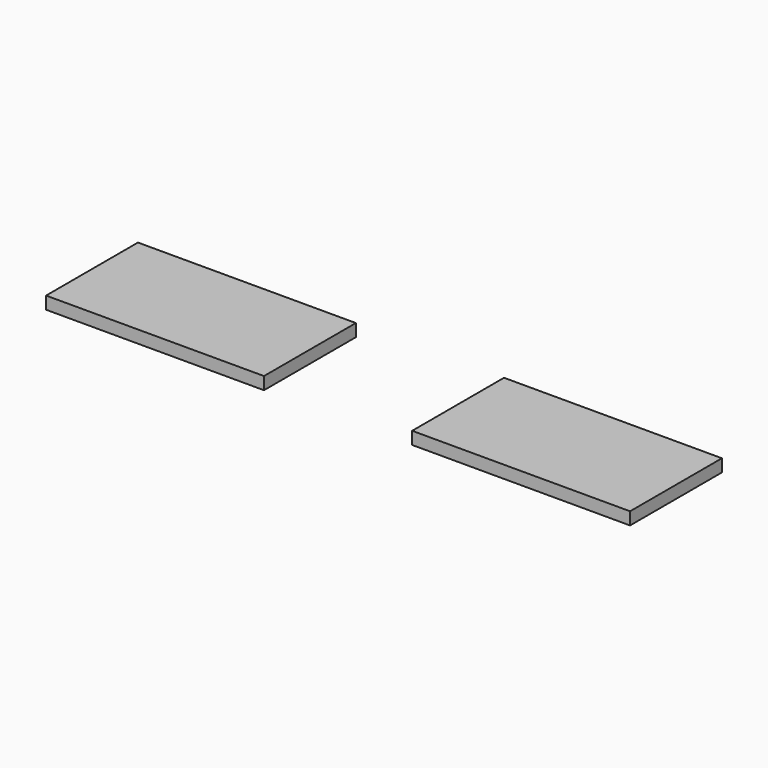
from build123d import *

# Parameters (mm, degrees)
F0_W     = 66.4195
F0_H     = 35
F1_DEPTH = 3.81


# Not quite as in the source:
# - a feature names something its author has since deleted; it is built from what else it names


with BuildPart() as f1:
    # F0 (on Top) → F1 (new body)
    with BuildSketch(Plane.XY):
        with Locations((-55.79025, 0)):
            Rectangle(F0_W, F0_H)
    extrude(amount=F1_DEPTH)


with BuildPart() as f1b:
    # F0 (on Top) → F1, piece 2 (new body)
    with BuildSketch(Plane.XY):
        with Locations((55.79025, 0)):
            Rectangle(F0_W, F0_H)
    extrude(amount=F1_DEPTH)


solid = Compound([f1.part, f1b.part])
